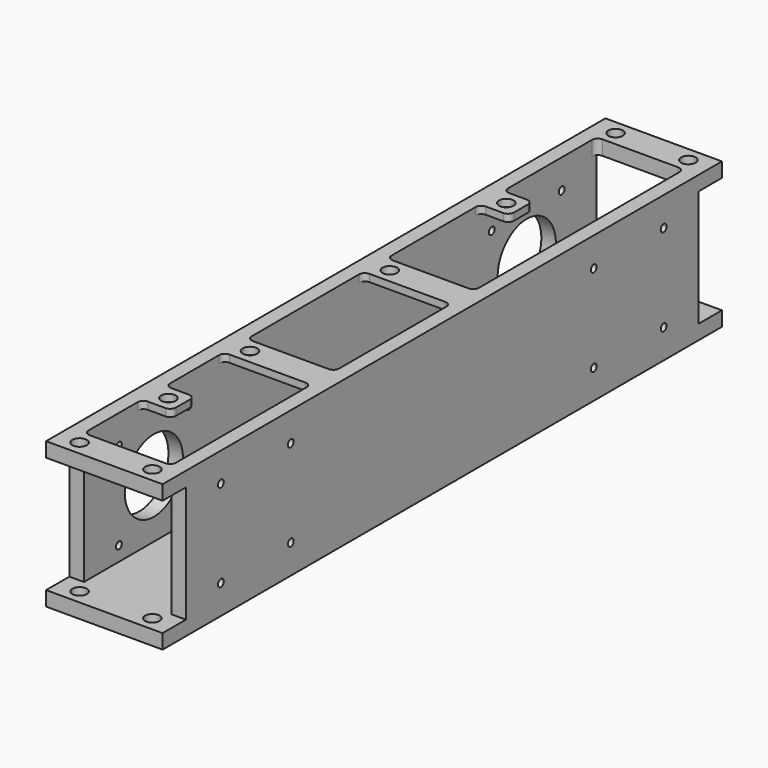
from build123d import *

# Parameters (mm, degrees)
F0_W      = 101.6
F0_H      = 609.6
F0_W_2    = 76.2
F0_H_2    = 558.8
F1_DEPTH  = 127
F2_W      = 76.2
F2_H      = 558.8
F3_DEPTH  = 19.05
F4_W      = 76.2
F4_H      = 25.4
F5_DEPTH  = 6.35
F6_W      = 101.6
F6_H      = 101.6
F7_DEPTH  = 25.4
F8_W      = 101.6
F8_H      = 101.6
F9_DEPTH  = 25.4
F10_DEPTH = 6.35
F11_R     = 6.35
F12_DEPTH = 6.35
F13_R     = 6.35
F14_DEPTH = 12.7
F15_DEPTH = 127
F16_W     = 25.4
F16_H     = 25.4
F17_DEPTH = 6.35
F18_R     = 6.35
F19_DEPTH = 6.35
F20_R     = 5.08
F21_R     = 31.75
F22_DEPTH = 12.7
F23_R     = 3.175
F24_DEPTH = 101.6


with BuildPart() as f1:
    # F0 (on Top) → F1 (new body)
    with BuildSketch(Plane.XY):
        with Locations((-88.1464483801, 27.3514616579)):
            Rectangle(F0_W, F0_H)
        with Locations((-88.1464483801, 27.3514616579)):
            Rectangle(F0_W_2, F0_H_2, mode=Mode.SUBTRACT)
    extrude(amount=F1_DEPTH)

    # F2 (on face) → F3 (join)
    with BuildSketch(Plane(origin=(0, 0, 0), x_dir=(1, 0, 0), z_dir=(0, 0, -1))):
        with Locations((-88.1464483801, -27.3514616579)):
            Rectangle(F2_W, F2_H)
    extrude(amount=-F3_DEPTH)

    # F4 (on face) → F5 (join)
    with BuildSketch(Plane.XY.offset(127)):
        with Locations((-88.1464483801, 65.4514616579)):
            Rectangle(F4_W, F4_H)
        with Locations((-88.1464483801, -86.9485383421)):
            Rectangle(F4_W, F4_H)
    extrude(amount=-F5_DEPTH)

    # F6 (on face) → F7 (cut)
    with BuildSketch(Plane.XZ.offset(277.4485383421)):
        with Locations((-88.1464483801, 63.5)):
            Rectangle(F6_W, F6_H)
    extrude(amount=-F7_DEPTH, mode=Mode.SUBTRACT)

    # F8 (on face) → F9 (cut)
    with BuildSketch(Plane(origin=(0, 332.1514616579, 0), x_dir=(-1, 0, 0), z_dir=(0, 1, 0))):
        with Locations((88.1464483801, 63.5)):
            Rectangle(F8_W, F8_H)
    extrude(amount=-F9_DEPTH, mode=Mode.SUBTRACT)

    # F10 (cut): a face of the model
    f10_faces = [f1.faces().sort_by_distance(p)[0] for p in [
        (-88.1464483801, 27.3514616579, 19.05),
    ]]
    extrude(f10_faces, amount=-F10_DEPTH, mode=Mode.SUBTRACT)

    # F11 (on face) → F12 (cut)
    with BuildSketch(Plane.XY.offset(127)):
        with Locations((-113.5464483801, 65.4514616579)):
            Circle(F11_R)
        with Locations((-113.5464483801, -86.9485383421)):
            Circle(F11_R)
    extrude(amount=-F12_DEPTH, mode=Mode.SUBTRACT)

    # F13 (on face) → F14 (cut)
    with BuildSketch(Plane.XY.offset(127)):
        with Locations((-119.8964483801, -264.7485383421)):
            Circle(F13_R)
        with Locations((-56.3964483801, -264.7485383421)):
            Circle(F13_R)
        with Locations((-119.8964483801, 319.4514616579)):
            Circle(F13_R)
        with Locations((-56.3964483801, 319.4514616579)):
            Circle(F13_R)
    extrude(amount=-F14_DEPTH, mode=Mode.SUBTRACT)

    # F13 (on face) → F15 (cut)
    with BuildSketch(Plane.XY.offset(127)):
        with Locations((-119.8964483801, 319.4514616579)):
            Circle(F13_R)
        with Locations((-56.3964483801, 319.4514616579)):
            Circle(F13_R)
        with Locations((-119.8964483801, -264.7485383421)):
            Circle(F13_R)
        with Locations((-56.3964483801, -264.7485383421)):
            Circle(F13_R)
    extrude(amount=-F15_DEPTH, mode=Mode.SUBTRACT)

    # F16 (on face) → F17 (join)
    with BuildSketch(Plane.XY.offset(127)):
        with Locations((-113.5464483801, -175.8485383421)):
            Rectangle(F16_W, F16_H)
        with Locations((-113.5464483801, 192.4514616579)):
            Rectangle(F16_W, F16_H)
    extrude(amount=-F17_DEPTH)

    # F18 (on face) → F19 (cut)
    with BuildSketch(Plane.XY.offset(127)):
        with Locations((-113.5464483801, 192.4514616579)):
            Circle(F18_R)
        with Locations((-113.5464483801, -175.8485383421)):
            Circle(F18_R)
    extrude(amount=-F19_DEPTH, mode=Mode.SUBTRACT)

    # F20
    f20_edges = [f1.edges().sort_by_distance(p)[0] for p in [
        (-126.246448, -99.648538, 123.825),
        (-50.046448, -99.648538, 123.825),
        (-100.846448, -163.148538, 123.825),
        (-100.846448, -188.548538, 123.825),
        (-126.246448, -188.548538, 123.825),
        (-126.246448, -163.148538, 123.825),
        (-50.046448, -252.048538, 120.65),
        (-50.046448, -74.248538, 123.825),
        (-126.246448, -74.248538, 123.825),
        (-50.046448, 52.751462, 123.825),
        (-126.246448, 52.751462, 123.825),
        (-126.246448, 179.751462, 123.825),
        (-126.246448, 78.151462, 123.825),
        (-50.046448, 78.151462, 123.825),
        (-100.846448, 179.751462, 123.825),
        (-126.246448, 205.151462, 123.825),
        (-100.846448, 205.151462, 123.825),
        (-126.246448, 306.751462, 120.65),
        (-126.246448, -252.048538, 120.65),
        (-50.046448, 306.751462, 120.65),
    ]]
    fillet(f20_edges, radius=F20_R)

    # F21 (on face) → F22 (cut)
    with BuildSketch(Plane(origin=(-138.9464483801, 0, 0), x_dir=(0, -1, 0), z_dir=(-1, 0, 0))):
        with Locations((-230.5514616579, 63.5)):
            Circle(F21_R)
        with Locations((175.8485383421, 63.5)):
            Circle(F21_R)
    extrude(amount=-F22_DEPTH, mode=Mode.SUBTRACT)

    # F23 (on face) → F24 (cut)
    with BuildSketch(Plane(origin=(-138.9464483801, 0, 0), x_dir=(0, -1, 0), z_dir=(-1, 0, 0))):
        with Locations((137.7485383421, 101.6)):
            Circle(F23_R)
        with Locations((137.7485383421, 25.4)):
            Circle(F23_R)
        with Locations((213.9485383421, 25.4)):
            Circle(F23_R)
        with Locations((213.9485383421, 101.6)):
            Circle(F23_R)
        with Locations((-192.4514616579, 25.4)):
            Circle(F23_R)
        with Locations((-268.6514616579, 25.4)):
            Circle(F23_R)
        with Locations((-268.6514616579, 101.6)):
            Circle(F23_R)
        with Locations((-192.4514616579, 101.6)):
            Circle(F23_R)
    extrude(amount=-F24_DEPTH, mode=Mode.SUBTRACT)


solid = f1.part
